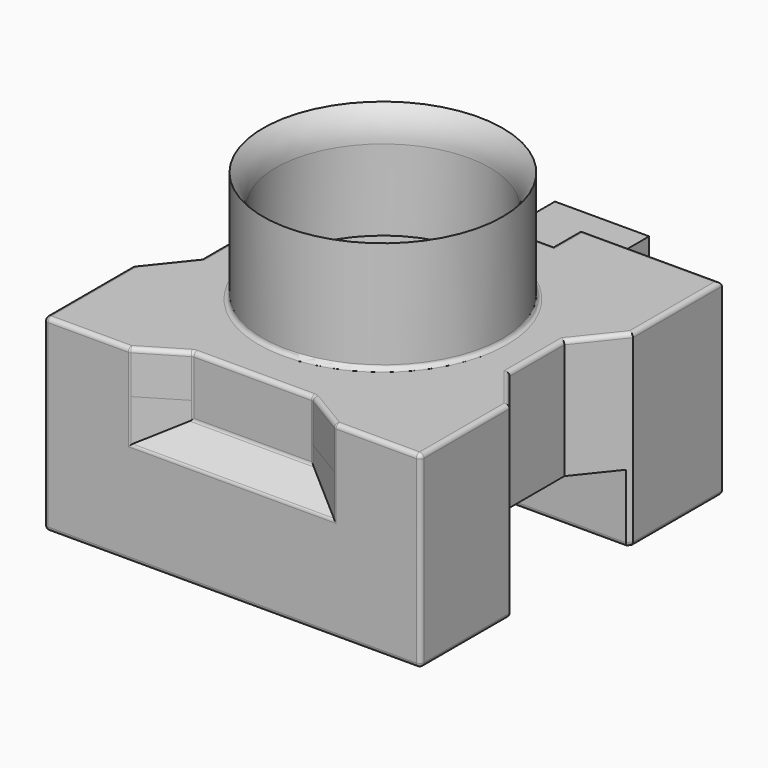
from build123d import *

# Parameters (mm, degrees)
F1_DEPTH    = 22
F2_DEPTH    = 17
F3_T4_DEPTH = 49.7168298797
F5_DEPTH    = 44
F0_W        = 11
F0_H        = 4
F6_DEPTH    = 15
F7_W        = 11
F7_H        = 2.2102209181
F8_DEPTH    = 14
F9_R        = 14
F9_R_2      = 12.5
F10_DEPTH   = 13
F12_R       = 0.5


# Not quite as in the source:
# - a fillet or chamfer that OpenCascade refuses, or shapes differently, is made with other operations: its cross-section is extruded or revolved along the edge and cut away or added


with BuildPart() as f1:
    # F0 (on Top) → F1 (new body)
    with BuildSketch(Plane.XY):
        Polygon((22, 9), (22, 22), (5.5, 22), (5.5, 18), (-5.5, 18), (-5.5, 22), (-22, 22), (-22, 9), (-18, 4), (-18, -4), (-22, -9), (-22, -22), (-12, -22), (-7, -19), (7, -19), (12, -22), (22, -22), (22, -9), (18, -4), (18, 4), align=None)
    extrude(amount=F1_DEPTH)

    # F0 (on Top) → F2 (join)
    with BuildSketch(Plane.XY):
        Polygon((-12, -22), (12, -22), (7, -19), (-7, -19), align=None)
    extrude(amount=F2_DEPTH)

    # F3: chamfer of 5 on 1 edges, made by hand


with BuildPart() as f3_tool2:
    # F3_s3 → F3_t4 (new body)
    with BuildSketch(Plane.YZ.offset(-24.8584149398)):
        Polygon((-17, 17), (-22, 12), (-22, 17), align=None)
    extrude(amount=F3_T4_DEPTH)

    split(bisect_by=Plane(origin=(-6.5294117647, -10.8823529412, 0), x_dir=(0, 0, 1), z_dir=(-0.5144957554, -0.8574929257, 0)), keep=Keep.TOP)

    split(bisect_by=Plane.XZ.offset(19), keep=Keep.TOP)

    split(bisect_by=Plane(origin=(6.5294117647, -10.8823529412, 0), x_dir=(0, 0, 1), z_dir=(0.5144957554, -0.8574929257, 0)), keep=Keep.TOP)


with BuildPart() as f1_1:
    add(f1.part)

    # F3_t1: cut F3_tool2
    add(f3_tool2.part, mode=Mode.SUBTRACT)

    # F4 (on face) → F5 (cut, through all)
    with BuildSketch(Plane.YZ.offset(22)):
        Polygon((8.5, 8), (-8.5, 8), (-8.5, 0), (0, 0), (8.5, 0), align=None)
    extrude(amount=-F5_DEPTH, mode=Mode.SUBTRACT)

    # F0 (on Top) → F6 (join)
    with BuildSketch(Plane.XY):
        with Locations((0, 20)):
            Rectangle(F0_W, F0_H)
    extrude(amount=F6_DEPTH)

    # F7 (on face) → F8 (join)
    with BuildSketch(Plane(origin=(0, 18, 0), x_dir=(-1, 0, 0), z_dir=(0, 1, 0))):
        with Locations((0, 16.105110459)):
            Rectangle(F7_W, F7_H)
    extrude(amount=F8_DEPTH)

    # F9 (on face) → F10 (join)
    with BuildSketch(Plane.XY.offset(22)):
        Circle(F9_R)
        Circle(F9_R_2, mode=Mode.SUBTRACT)
    extrude(amount=F10_DEPTH)

    # F11: fillet of radius 5 on 1 edges, made by hand

    # F11_s1 → F11_t2 (revolve, cut)
    with BuildSketch(Plane.XZ):
        with BuildLine():
            ThreePointArc((14, 35), (12.8902277714, 33.3657774588), (12.5, 31.4292857857))
            Line((12.5, 31.4292857857), (12.5, 35))
            Line((12.5, 35), (14, 35))
        make_face()
    revolve(axis=Axis((0, 0, 35), (0, 0, 1)), mode=Mode.SUBTRACT)

    # F12
    f12_edges = [f1_1.edges().sort_by_distance(p)[0] for p in [
        (22, 15.5, 22),
        (20, 6.5, 22),
        (13.75, 22, 22),
        (18, 0, 22),
        (5.5, 20, 22),
        (20, -6.5, 22),
        (0, 18, 22),
        (22, -15.5, 22),
        (-5.5, 20, 22),
        (17, -22, 22),
        (-13.75, 22, 22),
        (9.5, -20.5, 22),
        (-22, 15.5, 22),
        (0, -19, 22),
        (-20, 6.5, 22),
        (-9.5, -20.5, 22),
        (-18, 0, 22),
        (-17, -22, 22),
        (-20, -6.5, 22),
        (-22, -15.5, 22),
        (-14, 0, 22),
        (21.8, 8.75, 0),
        (22, 15.5, 0),
        (0, 22, 0),
        (-22, 15.5, 0),
        (-21.8, 8.75, 0),
        (0, 8.5, 0),
        (21.8, -8.75, 0),
        (22, -15.5, 0),
        (0, -22, 0),
        (-22, -15.5, 0),
        (-21.8, -8.75, 0),
        (0, -8.5, 0),
        (7, -19, 18.5),
        (0, -19, 15),
        (-7, -19, 18.5),
        (-22, -22, 11),
        (-12, -22, 17),
        (0, -22, 12),
        (12, -22, 17),
        (22, -22, 11),
        (-22, -9, 11),
    ]]
    fillet(f12_edges, radius=F12_R)


solid = f1_1.part
